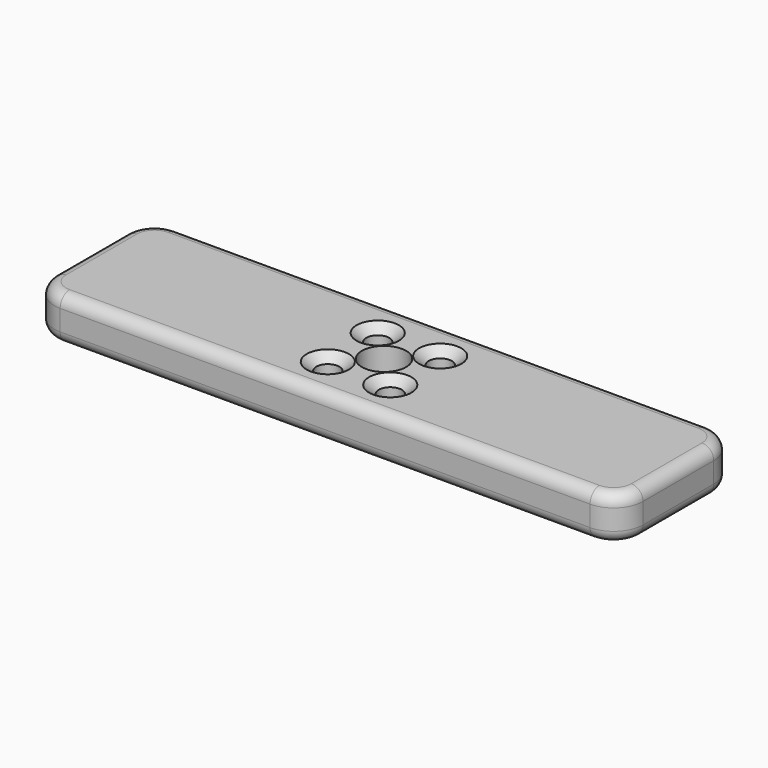
from build123d import *

# Parameters (mm, degrees)
F1_DEPTH        = 9.525
F2_R            = 2.54
F3_R            = 4.7625
F4_DEPTH        = 25.4
F6_D            = 4.9784
F6_CSINK_D      = 9.1186
F6_CSINK_ANGLE  = 100
F6_COPIES_COUNT = 4


# Not quite as in the source:
# - a pattern or mirror of a feature is missing from the dataset's text; its kind, count and spacing are read off the source's solid


with BuildPart() as f1:
    # F0 (on Top) → F1 (new body)
    with BuildSketch(Plane.XY):
        with BuildLine():
            Line((-57.15, -15.875), (57.15, -15.875))
            ThreePointArc((57.15, -15.875), (61.6401280605, -14.0151280605), (63.5, -9.525))
            Line((63.5, -9.525), (63.5, 9.525))
            ThreePointArc((63.5, 9.525), (61.6401280605, 14.0151280605), (57.15, 15.875))
            Line((57.15, 15.875), (-57.15, 15.875))
            ThreePointArc((-57.15, 15.875), (-61.6401280605, 14.0151280605), (-63.5, 9.525))
            Line((-63.5, 9.525), (-63.5, -9.525))
            ThreePointArc((-63.5, -9.525), (-61.6401280605, -14.0151280605), (-57.15, -15.875))
        make_face()
    extrude(amount=F1_DEPTH)

    # F2
    f2_edges = [f1.edges().sort_by_distance(p)[0] for p in [
        (0, -15.875, 9.525),
        (61.640128, -14.015128, 9.525),
        (63.5, 0, 9.525),
        (61.640128, 14.015128, 9.525),
        (0, 15.875, 9.525),
        (-61.640128, 14.015128, 9.525),
        (-63.5, 0, 9.525),
        (-61.640128, -14.015128, 9.525),
        (0, -15.875, 0),
        (61.640128, -14.015128, 0),
        (63.5, 0, 0),
        (61.640128, 14.015128, 0),
        (0, 15.875, 0),
        (-61.640128, 14.015128, 0),
        (-63.5, 0, 0),
        (-61.640128, -14.015128, 0),
    ]]
    fillet(f2_edges, radius=F2_R)

    # F3 (on face) → F4 (cut)
    with BuildSketch(Plane.XY.offset(9.525)):
        Circle(F3_R)
    extrude(amount=-F4_DEPTH, mode=Mode.SUBTRACT)

    # F6 (through all)
    with Locations(Plane.XY.offset(9.525)):
        with Locations((-6.7351920908, 6.7351920908)):
            f6 = CounterSinkHole(F6_D / 2, F6_CSINK_D / 2, counter_sink_angle=F6_CSINK_ANGLE)

    # F6_copies: F6 ×4 about axis
    f6_copies_axis = Axis((0, 0, 0), (0, 0, 1))
    for i in range(1, F6_COPIES_COUNT):
        add(f6.rotate(f6_copies_axis, i * 360 / F6_COPIES_COUNT), mode=Mode.SUBTRACT)


solid = f1.part
